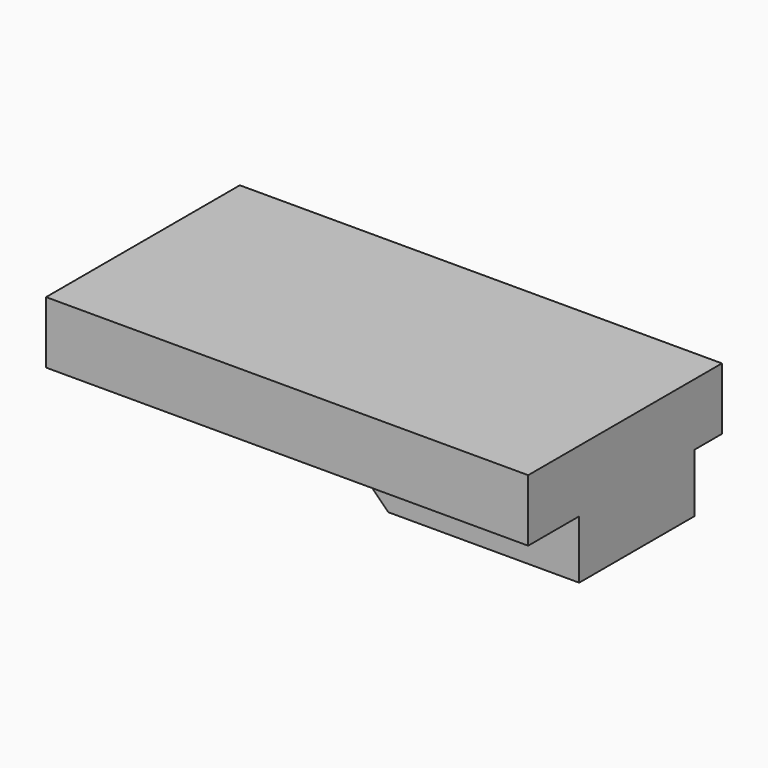
from build123d import *

# Parameters (mm, degrees)
F0_W        = 16.0388723016
F0_H        = 25.0722588971
F0_W_2      = 17.1450078487
F0_W_3      = 20.0946815312
F0_H_2      = 7.0054841926
F1_DEPTH    = 97.79
F2_W        = 83.8691648096
F2_H        = 58.0902062356
F4_DEPTH    = 23.622
F5_W        = 18.6321306974
F5_H        = 57.669268921
F6_DEPTH    = 23.622
F7_T4_DEPTH = 188.3107647097


# Not quite as in the source:
# - a fillet or chamfer that OpenCascade refuses, or shapes differently, is made with other operations: its cross-section is extruded or revolved along the edge and cut away or added


with BuildPart() as f1:
    # F0 (on Front) → F1 (new body)
    with BuildSketch(Plane.XZ):
        with Locations((-84.1579847038, 2.0279032178)):
            Rectangle(F0_W, F0_H)
        with Locations((93.9287915826, 2.0279032178)):
            Rectangle(F0_W_2, F0_H)
        Polygon((85.3562876582, 14.5640326664), (-76.138548553, 14.5640326664), (-76.138548553, -10.5082262307), (11.0612912104, -10.5082262307), (53.2785467803, -10.5082262307), (53.2785467803, -3.5027420381), (53.2785467803, 3.5027421545), (73.3732283115, 3.5027421545), (73.3732283115, -3.5027420381), (73.3732283115, -10.5082262307), (85.3562876582, -10.5082262307), align=None)
        with Locations((63.3258875459, 5.82e-08)):
            Rectangle(F0_W_3, F0_H_2)
        with Locations((63.3258875459, -7.0054841344)):
            Rectangle(F0_W_3, F0_H_2)
    extrude(amount=-F1_DEPTH)

    # F2 (on face) → F4 (join)
    with BuildSketch(Plane(origin=(0, 0, -10.5082262307), x_dir=(1, 0, 0), z_dir=(0, 0, -1))):
        with Locations((60.5667131022, -54.7835994512)):
            Rectangle(F2_W, F2_H)
    extrude(amount=F4_DEPTH)

    # F5 (on face) → F6 (join)
    with BuildSketch(Plane(origin=(0, 0, -10.5082262307), x_dir=(1, 0, 0), z_dir=(0, 0, -1))):
        with Locations((9.3160653487, -54.7836041078)):
            Rectangle(F5_W, F5_H)
    extrude(amount=F6_DEPTH)

    # F7: chamfer of 25.4 on 1 edges, made by hand


with BuildPart() as f7_tool2:
    # F7_s3 → F7_t4 (new body)
    with BuildSketch(Plane.XZ.offset(39.371778247)):
        Polygon((0, -8.7302262307), (25.4, -34.1302262307), (0, -34.1302262307), align=None)
    extrude(amount=-F7_T4_DEPTH)

    split(bisect_by=Plane.XY.offset(-10.5082262307), keep=Keep.BOTTOM)


with BuildPart() as f1_1:
    add(f1.part)

    # F7_t1: cut F7_tool2
    add(f7_tool2.part, mode=Mode.SUBTRACT)


solid = f1_1.part
